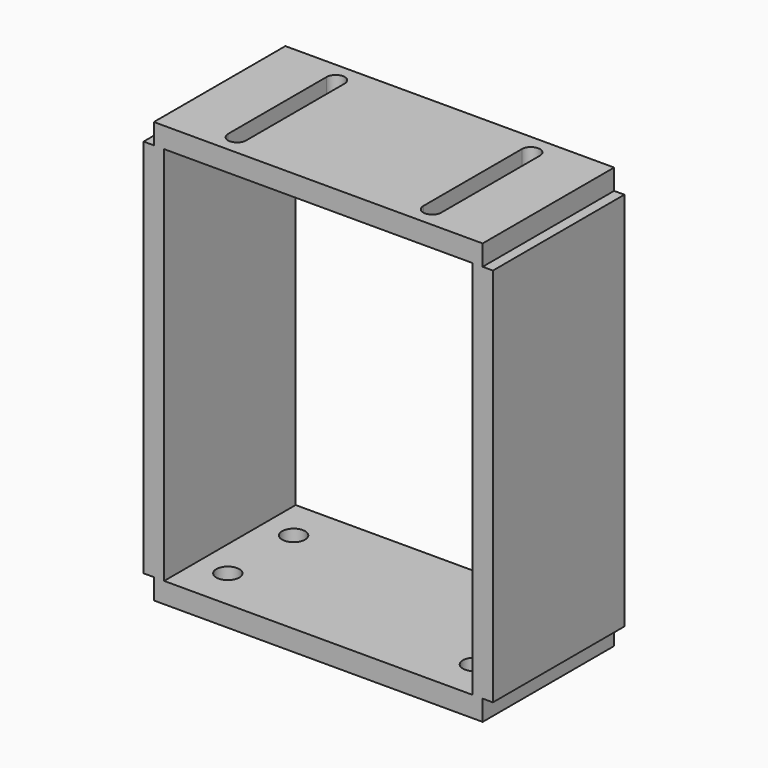
from build123d import *

# Parameters (mm, degrees)
F0_W     = 203.2
F0_H     = 101.6
F1_DEPTH = 12.7
F2_D     = 14.224
F4_W     = 203.2
F4_H     = 101.6
F5_DEPTH = 12.7
F7_DEPTH = 25.4
F8_W     = 101.6
F8_H     = 234.95
F9_DEPTH = 6.35


with BuildPart() as f1:
    # F0 (on Top) → F1 (new body)
    with BuildSketch(Plane.XY):
        Rectangle(F0_W, F0_H)
    extrude(amount=-F1_DEPTH)

    # F2 (through all)
    with Locations(Plane.XY):
        with Locations((-76.2, 25.4), (76.2, 25.4), (76.2, -25.4), (-76.2, -25.4)):
            Hole(F2_D / 2)



with BuildPart() as f5:
    # F4 (on offset) → F5 (new body)
    with BuildSketch(Plane(origin=(0, 0, 247.65), x_dir=(1, 0, 0), z_dir=(0, 0, -1))):
        Rectangle(F4_W, F4_H)
    extrude(amount=F5_DEPTH)

    # F6 (on face) → F7 (cut)
    with BuildSketch(Plane.XY.offset(247.65)):
        with BuildLine():
            Line((-54.76875, -12.7), (-54.76875, 12.7))
            ThreePointArc((-54.76875, 12.7), (-60.325, 7.14375), (-65.88125, 12.7))
            Line((-65.88125, 12.7), (-65.88125, -12.7))
            ThreePointArc((-65.88125, -12.7), (-60.325, -7.14375), (-54.76875, -12.7))
        make_face()
        with BuildLine():
            ThreePointArc((-65.88125, 12.7), (-60.325, 7.14375), (-54.76875, 12.7))
            Line((-54.76875, 12.7), (-54.76875, 38.1))
            ThreePointArc((-54.76875, 38.1), (-60.325, 43.65625), (-65.88125, 38.1))
            Line((-65.88125, 38.1), (-65.88125, 12.7))
        make_face()
        with BuildLine():
            Line((-54.76875, -38.1), (-54.76875, -12.7))
            ThreePointArc((-54.76875, -12.7), (-60.325, -7.14375), (-65.88125, -12.7))
            Line((-65.88125, -12.7), (-65.88125, -38.1))
            ThreePointArc((-65.88125, -38.1), (-60.325, -43.65625), (-54.76875, -38.1))
        make_face()
        with BuildLine():
            Line((54.76875, 12.7), (54.76875, -12.7))
            ThreePointArc((54.76875, -12.7), (60.325, -7.14375), (65.88125, -12.7))
            Line((65.88125, -12.7), (65.88125, 12.7))
            ThreePointArc((65.88125, 12.7), (60.325, 7.14375), (54.76875, 12.7))
        make_face()
        with BuildLine():
            ThreePointArc((65.88125, -12.7), (60.325, -7.14375), (54.76875, -12.7))
            Line((54.76875, -12.7), (54.76875, -38.1))
            ThreePointArc((54.76875, -38.1), (60.325, -43.65625), (65.88125, -38.1))
            Line((65.88125, -38.1), (65.88125, -12.7))
        make_face()
        with BuildLine():
            Line((54.76875, 38.1), (54.76875, 12.7))
            ThreePointArc((54.76875, 12.7), (60.325, 7.14375), (65.88125, 12.7))
            Line((65.88125, 12.7), (65.88125, 38.1))
            ThreePointArc((65.88125, 38.1), (60.325, 43.65625), (54.76875, 38.1))
        make_face()
    extrude(amount=-F7_DEPTH, mode=Mode.SUBTRACT)


with BuildPart() as f1_1:
    add(f1.part)

    add(f5.part)  # F9 merges F5
    # F8 (on face) → F9 (join, symmetric)
    with BuildSketch(Plane.YZ.offset(101.6)):
        with Locations((0, 117.475)):
            Rectangle(F8_W, F8_H)
    extrude(amount=F9_DEPTH, both=True)

    # F10: F1 across plane


with BuildPart() as f1_2:
    add(f1_1.part)
    add(f1_1.part.mirror(Plane.YZ))


solid = f1_2.part
